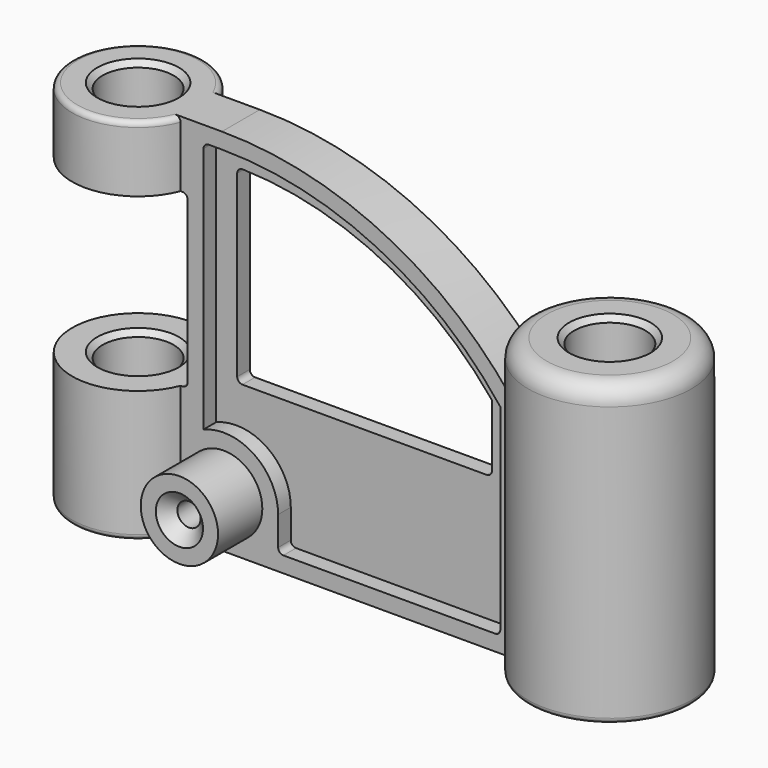
from build123d import *

# Parameters (mm, degrees)
F3_R            = 25
F4_DEPTH        = 140
F5_R            = 31
F6_DEPTH        = 113
F8_DEPTH        = 9
F9_R            = 13.5
F10_DEPTH       = 140
F12_R           = 2
F13_R           = 7
F14_SIZE        = 2
F15_R           = 14.668816826
F16_DEPTH       = 30
F18_DEPTH       = 6
F20_D           = 8.8
F20_CSINK_D     = 17.92
F20_CSINK_ANGLE = 90
F22_DEPTH       = 40.0010001
F24_DEPTH       = 31.0010001
F24_DEPTH_BACK  = 25
F25_SIZE        = 2


# Not quite as in the source:
# - a pattern or mirror of a feature is missing from the dataset's text; its kind, count and spacing are read off the source's solid


with BuildPart() as f4:
    # F3 (on Top) → F4 (new body)
    with BuildSketch(Plane.XY):
        Circle(F3_R)
    extrude(amount=F4_DEPTH)



with BuildPart() as f6:
    # F5 (on Top) → F6 (new body)
    with BuildSketch(Plane.XY):
        with Locations((179, 0)):
            Circle(F5_R)
    extrude(amount=F6_DEPTH)


with BuildPart() as f4_1:
    add(f4.part)

    add(f6.part)  # F8 merges F6
    # F7 (on Front) → F8 (join, symmetric)
    with BuildSketch(Plane.XZ):
        with BuildLine():
            Line((0, 0), (179, 0))
            ThreePointArc((179, 0), (137.9949493661, 98.9949493661), (39, 140))
            Line((39, 140), (0, 140))
            Line((0, 140), (0, 0))
        make_face()
    extrude(amount=F8_DEPTH, both=True)

    # F9 (on face) → F10 (cut, through all)
    with BuildSketch(Plane.XY.offset(140)):
        Circle(F9_R)
        with Locations((179, 0)):
            Circle(F9_R)
    extrude(amount=-F10_DEPTH, mode=Mode.SUBTRACT)

    # F12
    f12_edges = [f4_1.edges().sort_by_distance(p)[0] for p in [
        (-25, 0, 140),
        (-25, 0, 0),
        (183.549252, 30.664382, 0),
        (183.549252, -30.664382, 0),
    ]]
    fillet(f12_edges, radius=F12_R)

    # F13
    f13_edges = [f4_1.edges().sort_by_distance(p)[0] for p in [
        (148, 0, 113),
    ]]
    fillet(f13_edges, radius=F13_R)

    # F14
    f14_edges = [f4_1.edges().sort_by_distance(p)[0] for p in [
        (-13.5, 0, 140),
        (-13.5, 0, 0),
        (165.5, 0, 113),
        (165.5, 0, 0),
    ]]
    chamfer(f14_edges, length=F14_SIZE)

    # F15 (on Front) → F16 (join, symmetric)
    with BuildSketch(Plane.XZ):
        with Locations((39.6676030258, 19)):
            Circle(F15_R)
    extrude(amount=F16_DEPTH, both=True)

    # F17 (on face) → F18 (cut)
    with BuildSketch(Plane.XZ.offset(9)):
        with BuildLine():
            ThreePointArc((34, 134), (32.5857864376, 133.4142135624), (32, 132))
            Line((32, 132), (32, 38.1939535486))
            ThreePointArc((32, 38.1939535486), (51.2589728015, 36.1125724458), (60.3364198518, 19))
            Line((60.3364198518, 19), (60.3364198518, 8))
            ThreePointArc((60.3364198518, 8), (60.9222062895, 6.5857864376), (62.3364198518, 6))
            Line((62.3364198518, 6), (142.6676030258, 6))
            ThreePointArc((142.6676030258, 6), (144.0818165882, 6.5857864376), (144.6676030258, 8))
            Line((144.6676030258, 8), (144.6676030258, 82.4036265633))
            ThreePointArc((144.6676030258, 82.4036265633), (97.795892886, 120.411971912), (39, 134))
            Line((39, 134), (34, 134))
        make_face()
    f18 = extrude(amount=-F18_DEPTH, mode=Mode.SUBTRACT)

    # F18_copies: F18 across plane
    add(f18.mirror(Plane.ZX), mode=Mode.SUBTRACT)

    # F20 (through all)
    with Locations(Plane.XZ.offset(30)):
        with Locations((39.6676030258, 19)):
            CounterSinkHole(F20_D / 2, F20_CSINK_D / 2, counter_sink_angle=F20_CSINK_ANGLE)

    # F21 (on face) → F22 (cut, through all)
    with BuildSketch(Plane.XZ.offset(9)):
        with BuildLine():
            ThreePointArc((134.6676030258, 54), (136.0818165882, 54.5857864376), (136.6676030258, 56))
            Line((136.6676030258, 56), (136.6676030258, 79.6055231701))
            ThreePointArc((136.6676030258, 79.6055231701), (94.4363088441, 113.14952789), (42.0483870968, 125.963118952))
            ThreePointArc((42.0483870968, 125.963118952), (40.602998603, 125.3949231107), (40, 123.9637043654))
            Line((40, 123.9637043654), (40, 56))
            ThreePointArc((40, 56), (40.5857864376, 54.5857864376), (42, 54))
            Line((42, 54), (134.6676030258, 54))
        make_face()
    extrude(amount=-F22_DEPTH, mode=Mode.SUBTRACT)

    # F23 (on Front) → F24 (cut, two sides)
    with BuildSketch(Plane.XZ) as f24_sk:
        with BuildLine():
            Line((-34.1489688568, 115), (-34.1489688568, 50))
            Line((-34.1489688568, 50), (24, 50))
            ThreePointArc((24, 50), (25.4142135624, 50.5857864376), (26, 52))
            Line((26, 52), (26, 113))
            ThreePointArc((26, 113), (25.4142135624, 114.4142135624), (24, 115))
            Line((24, 115), (-34.1489688568, 115))
        make_face()
    extrude(amount=-F24_DEPTH, mode=Mode.SUBTRACT)
    extrude(f24_sk.sketch, amount=F24_DEPTH_BACK, mode=Mode.SUBTRACT)

    # F25
    f25_edges = [f4_1.edges().sort_by_distance(p)[0] for p in [
        (-13.5, 0, 50),
        (-13.5, 0, 115),
    ]]
    chamfer(f25_edges, length=F25_SIZE)


solid = f4_1.part
